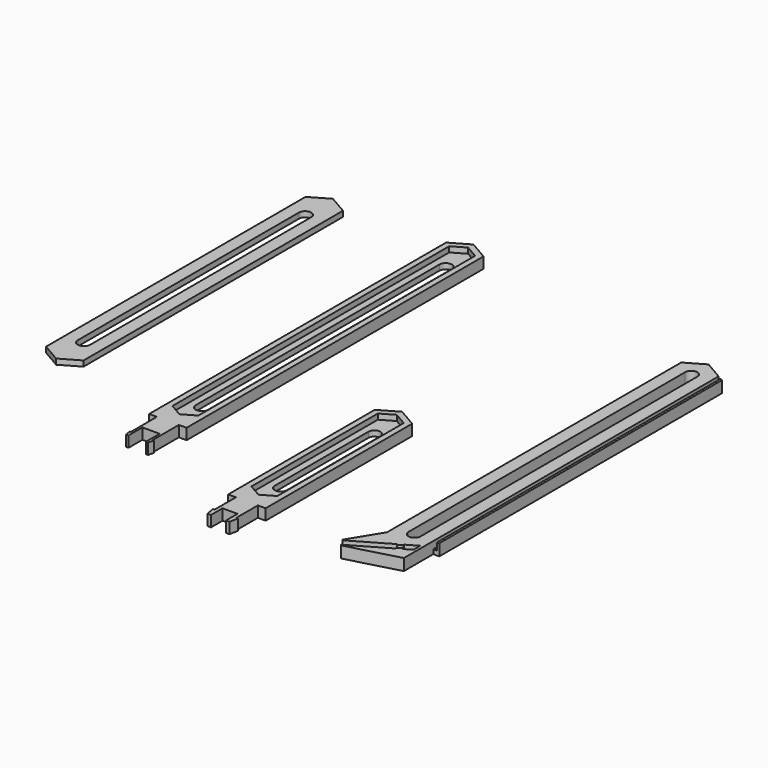
from build123d import *

# Parameters (mm, degrees)
F1_DEPTH = 1.9
F2_DEPTH = 1.9
F3_DEPTH = 4
F4_DEPTH = 1.5


# Not quite as in the source:
# - a feature names something its author has since deleted; it is built from what else it names


with BuildPart() as f1:
    # F0 (on Top) → F1 (new body, symmetric)
    with BuildSketch(Plane.XY):
        Polygon((-0.4, 2), (0, 0), (0.8, 0), (0.8, 6), (3.8, 6), (6.8, 6), (6.8, 0), (7.6, 0), (8, 2), (7.6, 2), (7.6, 13.3), (0, 13.3), (0, 2), align=None)
        Polygon((-2.7, 13.3), (0, 13.3), (7.6, 13.3), (10.3, 13.3), (10.3, 17.3), (-2.7, 17.3), align=None)
        Polygon((-2.7, 26.0947383738), (-2.7, 17.3), (10.3, 17.3), (10.3, 46.0942286341), (10.3, 135.7019237886), (10.3, 142.0527767497), (3.8, 145.8055534995), (-2.7, 142.0527767497), (-2.7, 135.7019237886), align=None)
        Polygon((8.3, 135.7019237886), (8.3, 26.0942286341), (8.3, 20.8980762114), (3.8, 18.3), (-0.7, 20.8980762114), (-0.7, 46.0947383738), (-0.7, 135.7019237886), (-0.7, 140.8980762114), (3.8, 143.4961524227), (8.3, 140.8980762114), align=None, mode=Mode.SUBTRACT)
    extrude(amount=F1_DEPTH, both=True)

    # F0 (on Top) → F2 (join)
    with BuildSketch(Plane.XY):
        Polygon((8.3, 20.8980762114), (8.3, 26.0942286341), (8.3, 135.7019237886), (8.3, 140.8980762114), (3.8, 143.4961524227), (-0.7, 140.8980762114), (-0.7, 135.7019237886), (-0.7, 46.0947383738), (-0.7, 20.8980762114), (3.8, 18.3), align=None)
        with BuildLine():
            ThreePointArc((5.95, 28.05), (3.8, 25.9), (1.65, 28.05))
            Line((1.65, 28.05), (1.65, 133.7461524227))
            ThreePointArc((1.65, 133.7461524227), (3.8, 135.8961524227), (5.95, 133.7461524227))
            Line((5.95, 133.7461524227), (5.95, 28.05))
        make_face(mode=Mode.SUBTRACT)
    extrude(amount=-F2_DEPTH)


with BuildPart() as f1b:
    # F0 (on Top) → F1, piece 2 (new body, symmetric)
    with BuildSketch(Plane.XY):
        Polygon((43.5, 24.8038475773), (43.5, -10.1961524227), (46.2, -10.1961524227), (46.2, -19.4961524227), (45.6, -19.4961524227), (46.2, -22.4961524227), (47.4, -22.4961524227), (47.4, -17.4961524227), (52.6, -17.4961524227), (52.6, -22.4961524227), (53.8, -22.4961524227), (54.4, -19.4961524227), (53.8, -19.4961524227), (53.8, -10.1961524227), (55.7, -10.1961524227), (56.5, -10.1961524227), (56.5, 24.8038475773), (56.5, 53.3604719043), (50, 57.1132486541), (43.5, 53.3604719043), align=None)
        Polygon((50, -5.1961524227), (45.5, -2.5980762114), (45.5, 2.5980762114), (45.5, 24.8038475773), (45.5, 47.0096189432), (45.5, 52.2057713659), (50, 54.8038475773), (54.5, 52.2057713659), (54.5, 47.0096189432), (54.5, 24.8038475773), (54.5, 2.5980762114), (54.5, -2.5980762114), align=None, mode=Mode.SUBTRACT)
    extrude(amount=F1_DEPTH, both=True)

    # F0 (on Top) → F2, piece 3 (join)
    with BuildSketch(Plane.XY):
        Polygon((45.5, 2.5980762114), (45.5, -2.5980762114), (50, -5.1961524227), (54.5, -2.5980762114), (54.5, 2.5980762114), (54.5, 24.8038475773), (54.5, 47.0096189432), (54.5, 52.2057713659), (50, 54.8038475773), (45.5, 52.2057713659), (45.5, 47.0096189432), (45.5, 24.8038475773), align=None)
        with BuildLine():
            ThreePointArc((52.1, 4.5038475773), (50, 2.4038475773), (47.9, 4.5038475773))
            Line((47.9, 4.5038475773), (47.9, 24.8038475773))
            Line((47.9, 24.8038475773), (47.9, 45.1038475773))
            ThreePointArc((47.9, 45.1038475773), (50, 47.2038475773), (52.1, 45.1038475773))
            Line((52.1, 45.1038475773), (52.1, 24.8038475773))
            Line((52.1, 24.8038475773), (52.1, 4.5038475773))
        make_face(mode=Mode.SUBTRACT)
    extrude(amount=-F2_DEPTH)


with BuildPart() as f2:
    # F0 (on Top) → F2, piece 2 (new body)
    with BuildSketch(Plane.XY):
        Polygon((-38.4546260238, 35.9091832103), (-38.4546260238, 85.8055534995), (-38.4546260238, 135.7019237886), (-38.4546260238, 142.0527767497), (-44.9546260238, 145.8055534995), (-51.4546260238, 142.0527767497), (-51.4546260238, 135.7019237886), (-51.4546260238, 85.8055534995), (-51.4546260238, 35.9091832103), (-51.4546260238, 29.5583302492), (-44.9546260238, 25.8055534995), (-38.4546260238, 29.5583302492), align=None)
        Polygon((-44.9546260238, 143.4961524227), (-40.4546260238, 140.8980762114), (-40.4546260238, 135.7019237886), (-40.4546260238, 85.8055534995), (-40.4546260238, 35.9091832103), (-40.4546260238, 30.7130307876), (-44.9546260238, 28.1149545762), (-49.4546260238, 30.7130307876), (-49.4546260238, 35.9091832103), (-49.4546260238, 85.8055534995), (-49.4546260238, 135.7019237886), (-49.4546260238, 140.8980762114), align=None, mode=Mode.SUBTRACT)
        Polygon((-40.4546260238, 135.7019237886), (-40.4546260238, 140.8980762114), (-44.9546260238, 143.4961524227), (-49.4546260238, 140.8980762114), (-49.4546260238, 135.7019237886), (-49.4546260238, 85.8055534995), (-49.4546260238, 35.9091832103), (-49.4546260238, 30.7130307876), (-44.9546260238, 28.1149545762), (-40.4546260238, 30.7130307876), (-40.4546260238, 35.9091832103), (-40.4546260238, 85.8055534995), align=None)
        with BuildLine():
            ThreePointArc((-47.1046260238, 133.7461524227), (-44.9546260238, 135.8961524227), (-42.8046260238, 133.7461524227))
            Line((-42.8046260238, 133.7461524227), (-42.8046260238, 85.8055534995))
            Line((-42.8046260238, 85.8055534995), (-42.8046260238, 37.8649545762))
            ThreePointArc((-42.8046260238, 37.8649545762), (-44.9546260238, 35.7149545762), (-47.1046260238, 37.8649545762))
            Line((-47.1046260238, 37.8649545762), (-47.1046260238, 85.8055534995))
            Line((-47.1046260238, 85.8055534995), (-47.1046260238, 133.7461524227))
        make_face(mode=Mode.SUBTRACT)
    extrude(amount=-F2_DEPTH)


with BuildPart() as f3:
    # F0 (on Top) → F3 (new body)
    with BuildSketch(Plane.XY):
        Polygon((93.5, 3.7527767497), (93.5, -3.7527767497), (100, -7.5055534995), (100.2, -7.851963661), (101.8019237886, -6.9270925304), (101.6019237886, -6.5806823689), (105.5, -4.3301270189), (105.5, -4.7920072343), (105.5, -6.7844546003), (105.5, -7.3323484187), (102.9019237886, -8.8323484187), (102.664678806, -8.4214280549), (101.0627550173, -9.3462991855), (101.3, -9.7572195493), (88.3096189432, -17.2572195493), (88.5096189432, -17.6036297108), (106.5, -12.7549981495), (106.5, -6.7549981495), (106.5, -6.2071043311), (106.5, -4.2146569651), (106.5, 0), (106.5, 3.7527767497), (106.5, 60), (106.5, 116.2472232503), (106.5, 123.7527767497), (100, 127.5055534995), (93.5, 123.7527767497), (93.5, 116.2472232503), (93.5, 60), align=None)
        with BuildLine():
            ThreePointArc((102.1, 0), (100, -2.1), (97.9, 0))
            Line((97.9, 0), (97.9, 60))
            Line((97.9, 60), (97.9, 120))
            ThreePointArc((97.9, 120), (100, 122.1), (102.1, 120))
            Line((102.1, 120), (102.1, 60))
            Line((102.1, 60), (102.1, 0))
        make_face(mode=Mode.SUBTRACT)
        Polygon((100, -7.5055534995), (93.5, -3.7527767497), (86.8096189432, -14.659143338), (87.0096189432, -15.0055534995), align=None)
    extrude(amount=F3_DEPTH)



with BuildPart() as f3b:
    # F0 (on Top) → F3, piece 2 (new body)
    with BuildSketch(Plane.XY):
        Polygon((108.6, 122.5403411844), (107.8, 123.0022213998), (107.8, 0), (108.6, 0), align=None)
    extrude(amount=F3_DEPTH)


with BuildPart() as f3_1:
    add(f3.part)

    add(f3b.part)  # F4 merges F3b
    # F0 (on Top) → F4 (join)
    with BuildSketch(Plane.XY):
        Polygon((107.8, 123.0022213998), (106.5, 123.7527767497), (106.5, 116.2472232503), (106.5, 60), (106.5, 3.7527767497), (106.5, 0), (107.8, 0), align=None)
        Polygon((100.2, -7.851963661), (100, -7.5055534995), (87.0096189432, -15.0055534995), (88.3096189432, -17.2572195493), (101.3, -9.7572195493), (101.0627550173, -9.3462991855), align=None)
    extrude(amount=F4_DEPTH)


solid = Compound([f1.part, f1b.part, f2.part, f3_1.part])
